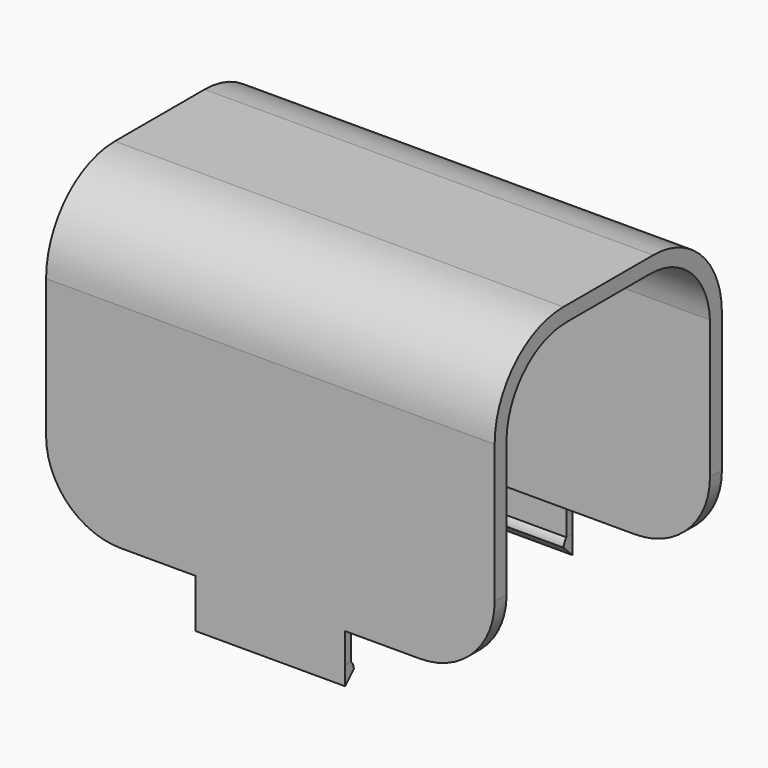
from build123d import *

# Parameters (mm, degrees)
F1_DEPTH     = 30
F2_R         = 10
F3_W         = 20
F3_H         = 1
F4_DEPTH     = 4
F6_DEPTH     = 3
F7_T1_DEPTH  = 26.6017443282
F8_T1_DEPTH  = 30.2743860668
F9_W         = 2
F9_H         = 3
F11_DEPTH    = 2
F10_W        = 2
F10_H        = 3
F12_DEPTH    = 2
F13_SIZE     = 1.99999
F14_T1_DEPTH = 10.6602829052
F14_T3_DEPTH = 10.6602829052


# Not quite as in the source:
# - a fillet or chamfer that OpenCascade refuses, or shapes differently, is made with other operations: its cross-section is extruded or revolved along the edge and cut away or added
# - a fillet or chamfer is up to 0.001 mm smaller than in the source, because OpenCascade refuses the exact size


with BuildPart() as f1:
    # F0 (on Right) → F1 (new body, symmetric)
    with BuildSketch(Plane.YZ):
        with BuildLine():
            Line((-2, 0), (0, 0))
            Line((0, 0), (0, 28.5))
            ThreePointArc((0, 28.5), (-3.3682720164, 36.6317279836), (-11.5, 40))
            Line((-11.5, 40), (-26.5, 40))
            ThreePointArc((-26.5, 40), (-34.6317279836, 36.6317279836), (-38, 28.5))
            Line((-38, 28.5), (-38, 0))
            Line((-38, 0), (-36, 0))
            Line((-36, 0), (-36, 28.5))
            ThreePointArc((-36, 28.5), (-32.9045321983, 35.2456883731), (-26.0125078223, 38))
            Line((-26.0125078223, 38), (-11.9874921777, 38))
            ThreePointArc((-11.9874921777, 38), (-5.0954678017, 35.2456883731), (-2, 28.5))
            Line((-2, 28.5), (-2, 0))
        make_face()
    extrude(amount=F1_DEPTH, both=True)

    # F2
    f2_edges = [f1.edges().sort_by_distance(p)[0] for p in [
        (30, -37, 0),
        (30, -1, 0),
        (-30, -1, 0),
        (-30, -37, 0),
    ]]
    fillet(f2_edges, radius=F2_R)

    # F3 (on face) → F4 (join)
    with BuildSketch(Plane(origin=(0, 0, 0), x_dir=(1, 0, 0), z_dir=(0, 0, -1))):
        with Locations((0, 0.5)):
            Rectangle(F3_W, F3_H)
        with Locations((0, 37.5)):
            Rectangle(F3_W, F3_H)
    extrude(amount=F4_DEPTH)

    # F5 (on face) → F6 (join)
    with BuildSketch(Plane(origin=(0, 0, -4), x_dir=(1, 0, 0), z_dir=(0, 0, -1))):
        Polygon((10, 38), (-10, 38), (-10, 36.5000508078), (9.987654115, 36.5000508078), align=None)
        Polygon((-10, 1.4999491922), (-10, 0), (10, 0), (9.987654115, 1.4999491922), align=None)
    extrude(amount=F6_DEPTH)

    # F7: fillet of radius 2 on 2 edges, made by hand

    # F7_s2 → F7_t1 (cut)
    with BuildSketch(Plane.YZ.offset(-13.3070451066)):
        with BuildLine():
            ThreePointArc((-1.4999491922, -5.3228180426), (-1.3707914645, -4.6157471889), (-1, -4))
            Line((-1, -4), (-1.4999491922, -4))
            Line((-1.4999491922, -4), (-1.4999491922, -5.3228180426))
        make_face()
        with BuildLine():
            ThreePointArc((-37, -4), (-36.6292085355, -4.6157471889), (-36.5000508078, -5.3228180426))
            Line((-36.5000508078, -5.3228180426), (-36.5000508078, -4))
            Line((-36.5000508078, -4), (-37, -4))
        make_face()
    extrude(amount=F7_T1_DEPTH, mode=Mode.SUBTRACT)

    # F8: chamfer of 2 on 2 edges, made by hand

    # F8_s2 → F8_t1 (cut)
    with BuildSketch(Plane.YZ.offset(-15.1433659759)):
        Polygon((0.5000508078, -7), (-1.4999491922, -5), (-1.4999491922, -7), align=None)
        Polygon((-38.5000508078, -7), (-36.5000508078, -5), (-36.5000508078, -7), align=None)
    extrude(amount=F8_T1_DEPTH, mode=Mode.SUBTRACT)

    # F9 (on face) → F11 (join)
    with BuildSketch(Plane.XZ.offset(2)):
        Polygon((-25, 11), (-25, 10), (-25, 9), (-22, 9), (-22, 11), align=None)
        with Locations((-23.5, 14.5)):
            Rectangle(F9_W, F9_H)
        Polygon((-5, 9), (-5, 10), (-5, 11), (-8, 11), (-8, 9), align=None)
        with Locations((-6.5, 14.5)):
            Rectangle(F9_W, F9_H)
    extrude(amount=F11_DEPTH)

    # F10 (on face) → F12 (join)
    with BuildSketch(Plane(origin=(0, -36, 0), x_dir=(-1, 0, 0), z_dir=(0, 1, 0))):
        Polygon((22, 11), (22, 10), (22, 9), (25, 9), (25, 11), align=None)
        with Locations((23.5, 14.5)):
            Rectangle(F10_W, F10_H)
        Polygon((8, 9), (8, 10), (8, 11), (5, 11), (5, 9), align=None)
        with Locations((6.5, 14.5)):
            Rectangle(F10_W, F10_H)
    extrude(amount=F12_DEPTH)

    # F13 (size 2 in the source; OpenCascade refuses exactly that, so slightly less here)
    f13_edges = [f1.edges().sort_by_distance(p)[0] for p in [
        (-23.5, -4, 16),
        (-23.5, -34, 16),
        (-6.5, -4, 16),
        (-6.5, -34, 16),
    ]]
    chamfer(f13_edges, length=F13_SIZE)

    # F14: fillet of radius 2 on 4 edges, made by hand

    # F14_s2 → F14_t1 (cut)
    with BuildSketch(Plane.YZ.offset(-28.8301414526)):
        with BuildLine():
            ThreePointArc((-4, 14.00001), (-3.267948419, 13.2679520792), (-2.267943419, 13))
            Line((-2.267943419, 13), (-4, 13))
            Line((-4, 13), (-4, 14.00001))
        make_face()
        with BuildLine():
            ThreePointArc((-35.732056581, 13), (-34.732051581, 13.2679520792), (-34, 14.00001))
            Line((-34, 14.00001), (-34, 13))
            Line((-34, 13), (-35.732056581, 13))
        make_face()
    extrude(amount=F14_T1_DEPTH, mode=Mode.SUBTRACT)

    # F14_s4 → F14_t3 (cut)
    with BuildSketch(Plane.YZ.offset(-11.8301414526)):
        with BuildLine():
            ThreePointArc((-2.267943419, 13), (-3.267948419, 13.2679520792), (-4, 14.00001))
            Line((-4, 14.00001), (-4, 13))
            Line((-4, 13), (-2.267943419, 13))
        make_face()
        with BuildLine():
            ThreePointArc((-35.732056581, 13), (-34.732051581, 13.2679520792), (-34, 14.00001))
            Line((-34, 14.00001), (-34, 13))
            Line((-34, 13), (-35.732056581, 13))
        make_face()
    extrude(amount=F14_T3_DEPTH, mode=Mode.SUBTRACT)


solid = f1.part
